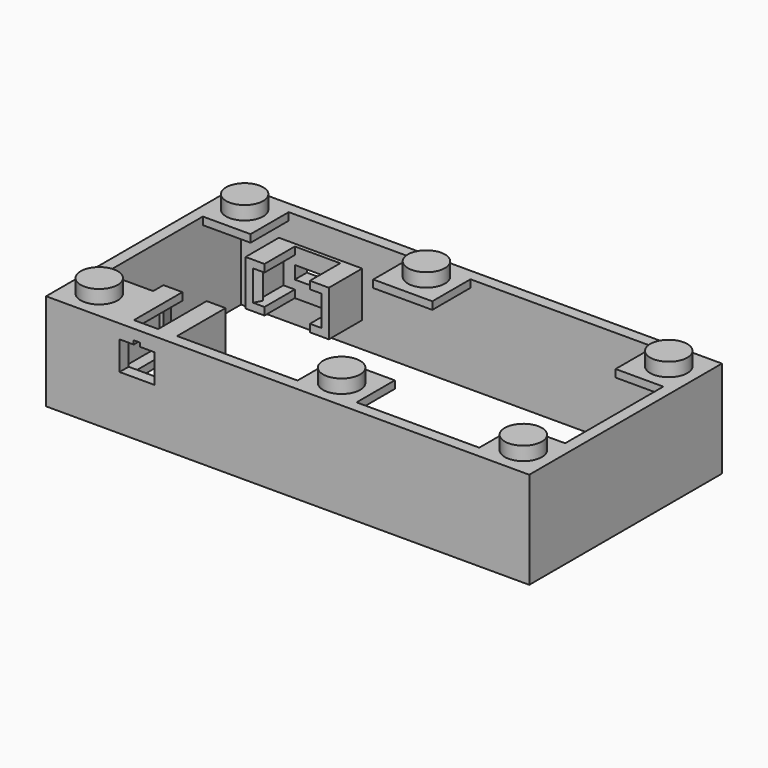
from build123d import *

# Parameters (mm, degrees)
F0_W      = 63.8
F0_H      = 31.8
F0_W_2    = 60.8
F0_H_2    = 28.8
F1_DEPTH  = 12.8
F2_W      = 6.3
F2_H      = 6.3
F2_W_2    = 7.8
F3_DEPTH  = 1
F4_R      = 2.45
F5_DEPTH  = 1.8
F6_W      = 0.85
F6_H      = 0.5
F7_DEPTH  = 25.4
F9_DEPTH  = 8
F11_DEPTH = 5
F12_W     = 0.1
F12_H     = 1
F13_DEPTH = 6.3
F14_W     = 6
F14_H     = 1.7
F15_DEPTH = 2.54
F16_W     = 11
F16_H     = 6
F16_W_2   = 6
F16_H_2   = 1.7
F17_DEPTH = 0.5
F19_DEPTH = 5
F21_DEPTH = 4


# Not quite as in the source:
# - a feature names something its author has since deleted; it is built from what else it names


with BuildPart() as f1:
    # F0 (on Top) → F1 (new body)
    with BuildSketch(Plane.XY):
        with Locations((31.9, 15.9)):
            Rectangle(F0_W, F0_H)
        with Locations((31.9, 15.9)):
            Rectangle(F0_W_2, F0_H_2, mode=Mode.SUBTRACT)
    extrude(amount=F1_DEPTH)

    # F2 (on face) → F3 (join)
    with BuildSketch(Plane.XY.offset(12.8)):
        with Locations((4.65, 27.15)):
            Rectangle(F2_W, F2_H)
        with Locations((4.65, 4.65)):
            Rectangle(F2_W, F2_H)
        with Locations((59.15, 4.65)):
            Rectangle(F2_W, F2_H)
        with Locations((59.15, 27.15)):
            Rectangle(F2_W, F2_H)
        with Locations((27.9, 27.15)):
            Rectangle(F2_W_2, F2_H)
        with Locations((35.9, 4.65)):
            Rectangle(F2_W_2, F2_H)
    extrude(amount=-F3_DEPTH)

    # F4 (on face) → F5 (join)
    with BuildSketch(Plane.XY.offset(12.8)):
        with Locations((3.9, 27.9)):
            Circle(F4_R)
        with Locations((59.9, 27.9)):
            Circle(F4_R)
        with Locations((59.9, 3.9)):
            Circle(F4_R)
        with Locations((3.9, 3.9)):
            Circle(F4_R)
        with Locations((27.9, 27.9)):
            Circle(F4_R)
        with Locations((35.9, 3.9)):
            Circle(F4_R)
    extrude(amount=F5_DEPTH)

    # F6 (on face) → F7 (cut)
    with BuildSketch(Plane.XZ):
        Polygon((11.575, 10.95), (9.7, 10.95), (9.7, 7.15), (14.3, 7.15), (14.3, 10.95), (12.425, 10.95), align=None)
        with Locations((12, 11.2)):
            Rectangle(F6_W, F6_H)
    extrude(amount=-F7_DEPTH, mode=Mode.SUBTRACT)

    # F8 (on face) → F9 (join)
    with BuildSketch(Plane(origin=(0, 1.5, 0), x_dir=(-1, 0, 0), z_dir=(0, 1, 0))):
        Polygon((-13.6, 5.8), (-13.6, 6.8), (-15.1, 6.8), (-15.1, 11.8), (-13.6, 11.8), (-13.6, 12.8), (-16.1, 12.8), (-16.1, 5.8), align=None)
        Polygon((-8.9, 6.8), (-10.4, 6.8), (-10.4, 5.8), (-7.9, 5.8), (-7.9, 12.8), (-10.4, 12.8), (-10.4, 11.8), (-8.9, 11.8), align=None)
    extrude(amount=F9_DEPTH)

    # F10 (on face) → F11 (join, through all)
    with BuildSketch(Plane.XY.offset(6.8)):
        Polygon((14.6, 7.6), (15.1, 7.6), (15.1, 9.5), align=None)
        Polygon((9.4, 7.6), (8.9, 9.5), (8.9, 7.6), align=None)
    extrude(amount=F11_DEPTH)

    # F12 (on face) → F13 (join, through all)
    with BuildSketch(Plane(origin=(0, 1.5, 0), x_dir=(-1, 0, 0), z_dir=(0, 1, 0))):
        with Locations((-7.85, 12.3)):
            Rectangle(F12_W, F12_H)
    extrude(amount=F13_DEPTH)

    # F14 (on face) → F15 (cut)
    with BuildSketch(Plane(origin=(0, 31.8, 0), x_dir=(-1, 0, 0), z_dir=(0, 1, 0))):
        with Locations((-12, 6.4)):
            Rectangle(F14_W, F14_H)
    extrude(amount=-F15_DEPTH, mode=Mode.SUBTRACT)

    # F16 (on face) → F17 (join)
    with BuildSketch(Plane.XZ.offset(-30.3)):
        with Locations((12, 6.4)):
            Rectangle(F16_W, F16_H)
        with Locations((12, 6.4)):
            Rectangle(F16_W_2, F16_H_2, mode=Mode.SUBTRACT)
    extrude(amount=F17_DEPTH)

    # F18 (on face) → F19 (join)
    with BuildSketch(Plane.XZ.offset(-29.8)):
        Polygon((9, 9.4), (6.5, 9.4), (6.5, 3.4), (9, 3.4), (9, 4.4), (7.5, 4.4), (7.5, 8.4), (9, 8.4), align=None)
        Polygon((17.5, 9.4), (15, 9.4), (15, 8.4), (16.5, 8.4), (16.5, 4.4), (15, 4.4), (15, 3.4), (17.5, 3.4), align=None)
    extrude(amount=F19_DEPTH)

    # F20 (on face) → F21 (join, through all)
    with BuildSketch(Plane.XY.offset(4.4)):
        Polygon((7.5, 25.8), (7.5, 24.8), (8, 25.8), align=None)
        Polygon((16, 25.8), (16.5, 24.8), (16.5, 25.8), align=None)
    extrude(amount=F21_DEPTH)


solid = f1.part
